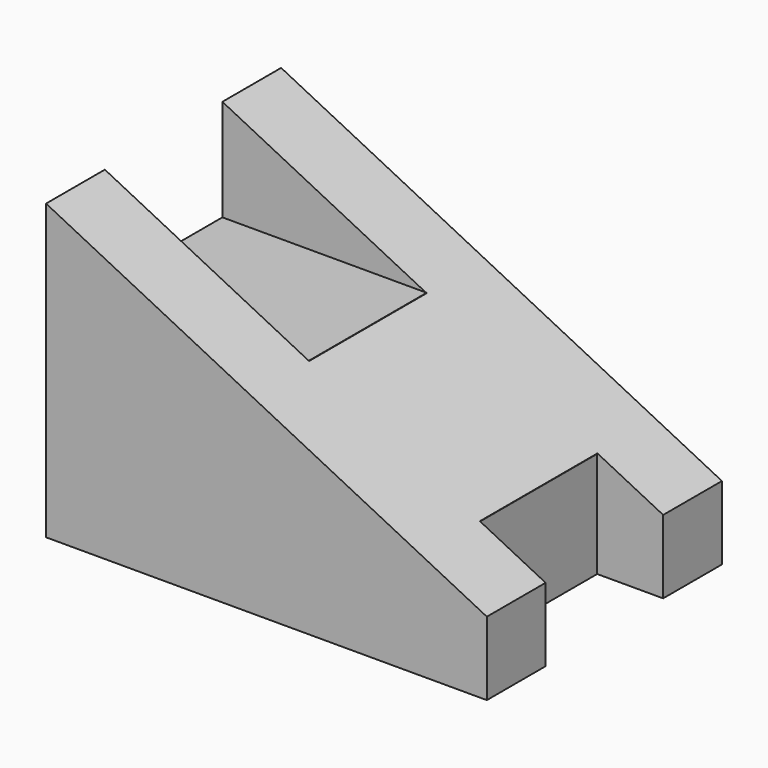
from build123d import *

# Parameters (mm, degrees)
F1_DEPTH  = 20
F2_W      = 10
F2_H      = 5
F3_DEPTH  = 5
F4_W      = 5
F4_H      = 10
F5_DEPTH  = 15
F6_W      = 15.5
F6_H      = 10
F7_DEPTH  = 7.5
F8_W      = 3.6006319447
F8_H      = 10
F9_DEPTH  = 7.2
F10_W     = 10
F10_H     = 1.4608040711
F11_DEPTH = 13.9


with BuildPart() as f1:
    # F0 (on Front) → F1 (new body)
    with BuildSketch(Plane.XZ):
        Polygon((0, 20), (0, 0), (30, 0), (30, 5), align=None)
    extrude(amount=F1_DEPTH)

    # F2 (on face) → F3 (cut)
    with BuildSketch(Plane.YZ.offset(30)):
        with Locations((-10, 2.5)):
            Rectangle(F2_W, F2_H)
    extrude(amount=-F3_DEPTH, mode=Mode.SUBTRACT)

    # F4 (on face) → F5 (cut)
    with BuildSketch(Plane(origin=(8, 0, 16), x_dir=(0.894427191, 0, -0.4472135955), z_dir=(0.4472135955, 0, 0.894427191))):
        with Locations((22.0967477525, -10)):
            Rectangle(F4_W, F4_H)
    extrude(amount=-F5_DEPTH, mode=Mode.SUBTRACT)

    # F6 (on face) → F7 (cut)
    with BuildSketch(Plane(origin=(8, 0, 16), x_dir=(0.894427191, 0, -0.4472135955), z_dir=(0.4472135955, 0, 0.894427191))):
        with Locations((-1.19427191, -10)):
            Rectangle(F6_W, F6_H)
    extrude(amount=-F7_DEPTH, mode=Mode.SUBTRACT)

    # F8 (on face) → F9 (join)
    with BuildSketch(Plane(origin=(0, 0, 0), x_dir=(1, 0, 0), z_dir=(0, 0, -1))):
        with Locations((23.7101460286, 10)):
            Rectangle(F8_W, F8_H)
    extrude(amount=-F9_DEPTH)


with BuildPart() as f11:
    # F10 (on face) → F11 (new body)
    with BuildSketch(Plane(origin=(0, 0, 0), x_dir=(0, -1, 0), z_dir=(-1, 0, 0))):
        with Locations((10, 12.3451471199)):
            Rectangle(F10_W, F10_H)
    extrude(amount=-F11_DEPTH)


solid = Compound([f1.part, f11.part])
